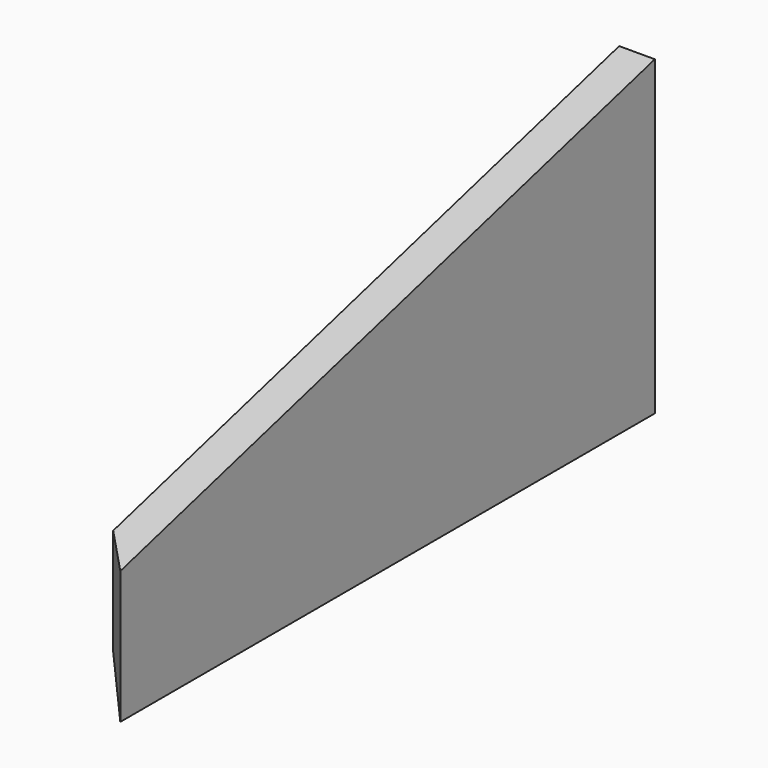
from build123d import *

# Parameters (mm, degrees)
F1_DEPTH = 16
F2_SIZE  = 15.99999


# Not quite as in the source:
# - a fillet or chamfer is up to 0.001 mm smaller than in the source, because OpenCascade refuses the exact size


with BuildPart() as f1:
    # F0 (on Right) → F1 (new body)
    with BuildSketch(Plane.YZ):
        Polygon((0, 59.6152422707), (0, 0), (300, 0), (300, 140), align=None)
    extrude(amount=F1_DEPTH)

    # F2 (size 16 in the source; OpenCascade refuses exactly that, so slightly less here)
    f2_edges = [f1.edges().sort_by_distance(p)[0] for p in [
        (0, 0, 29.807621),
        (0, 150, 0),
    ]]
    chamfer(f2_edges, length=F2_SIZE)


solid = f1.part
